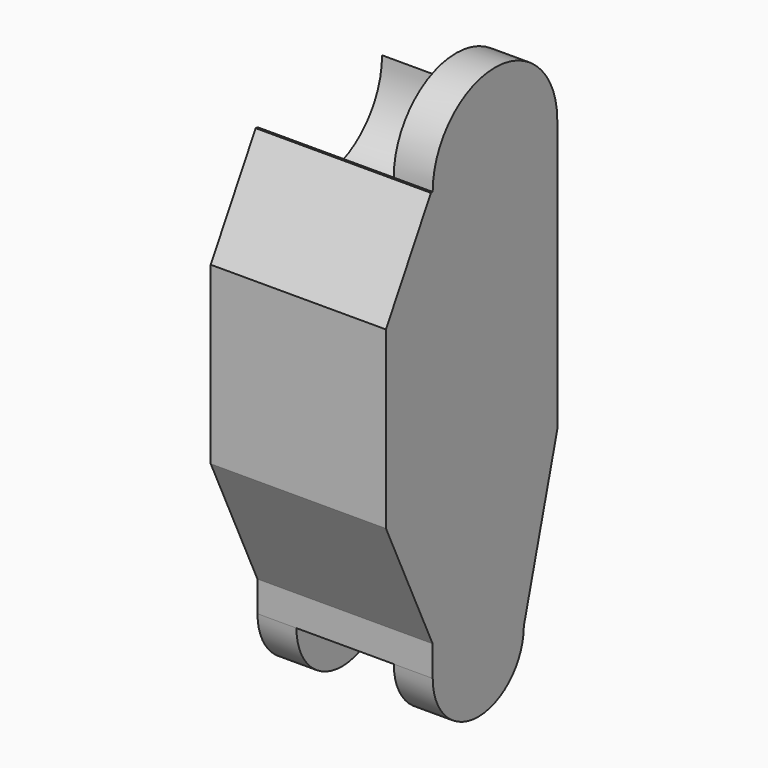
from build123d import *

# Parameters (mm, degrees)
F1_DEPTH     = 19.05
F2_DEPTH     = 114.3
F3_W         = 114.3
F3_H         = 101.6
F4_DEPTH     = 177.8
F5_T1_DEPTH  = 641.9538230647
F6_R         = 37.1475
F7_DEPTH     = 25.4
F8_R         = 37.1475
F9_DEPTH     = 25.4
F10_W        = 114.3
F10_H        = 266.7
F11_DEPTH    = 38.1
F12_T4_DEPTH = 574.9754388191
F13_T1_DEPTH = 442.85989084
F14_START    = 88.9
F14_DEPTH    = 25.4


# Not quite as in the source:
# - a fillet or chamfer that OpenCascade refuses, or shapes differently, is made with other operations: its cross-section is extruded or revolved along the edge and cut away or added


with BuildPart() as f1:
    # F0 (on Right) → F1 (new body)
    with BuildSketch(Plane.YZ):
        with BuildLine():
            Line((50.8, -101.6), (50.8, 0))
            ThreePointArc((50.8, 0), (0, -50.8), (-50.8, 0))
            Line((-50.8, 0), (-50.8, -101.6))
            Line((-50.8, -101.6), (50.8, -101.6))
        make_face()
    extrude(amount=F1_DEPTH)

    # F0 (on Right) → F2 (join)
    with BuildSketch(Plane.YZ):
        with BuildLine():
            Line((50.8, -101.6), (50.8, 0))
            ThreePointArc((50.8, 0), (0, -50.8), (-50.8, 0))
            Line((-50.8, 0), (-50.8, -101.6))
            Line((-50.8, -101.6), (50.8, -101.6))
        make_face()
    extrude(amount=F2_DEPTH)

    # F3 (on face) → F4 (join)
    with BuildSketch(Plane(origin=(0, 0, -101.6), x_dir=(1, 0, 0), z_dir=(0, 0, -1))):
        with Locations((57.15, 0)):
            Rectangle(F3_W, F3_H)
    extrude(amount=F4_DEPTH)

    # F5: chamfer of 101.6 x 27.223637951 on 1 edges, made by hand

    # F5_s2 → F5_t1 (cut)
    with BuildSketch(Plane.YZ.offset(-263.8269115324)):
        Polygon((23.576362049, -279.4), (50.8, -177.8), (50.8, -279.4), align=None)
    extrude(amount=F5_T1_DEPTH, mode=Mode.SUBTRACT)

    # F6 (on face) → F7 (join)
    with BuildSketch(Plane(origin=(0, 0, 0), x_dir=(0, -1, 0), z_dir=(-1, 0, 0))):
        with Locations((13.6118189755, -279.4)):
            Circle(F6_R)
    extrude(amount=-F7_DEPTH)

    # F8 (on face) → F9 (join)
    with BuildSketch(Plane.YZ.offset(114.3)):
        with Locations((-13.6118189755, -279.4)):
            Circle(F8_R)
    extrude(amount=-F9_DEPTH)

    # F10 (on face) → F11 (join)
    with BuildSketch(Plane.XZ.offset(50.8)):
        with Locations((57.15, -133.35)):
            Rectangle(F10_W, F10_H)
    extrude(amount=F11_DEPTH)

    # F12: chamfer of 88.9 x 41.45475081 on 1 edges, made by hand


with BuildPart() as f12_tool2:
    # F12_s3 → F12_t4 (new body)
    with BuildSketch(Plane.YZ.offset(-230.3377194096)):
        Polygon((-88.9, -177.8), (-47.44524919, -266.7), (-88.9, -266.7), align=None)
    extrude(amount=F12_T4_DEPTH)

    split(bisect_by=Plane.XZ.offset(50.8), keep=Keep.TOP)


with BuildPart() as f1_1:
    add(f1.part)

    # F12_t1: cut F12_tool2
    add(f12_tool2.part, mode=Mode.SUBTRACT)

    # F13: chamfer of 63.5 x 36.6617420935 on 1 edges, made by hand

    # F13_s2 → F13_t1 (cut)
    with BuildSketch(Plane.YZ.offset(-164.27994542)):
        Polygon((-88.9, -63.5), (-52.2382579065, 0), (-88.9, 0), align=None)
    extrude(amount=F13_T1_DEPTH, mode=Mode.SUBTRACT)

    # F0 (on Right) → F14 (join)
    with BuildSketch(Plane.YZ.offset(F14_START)):
        with BuildLine():
            Line((-50.8, 0), (50.8, 0))
            ThreePointArc((50.8, 0), (0, 50.8), (-50.8, 0))
        make_face()
        with BuildLine():
            ThreePointArc((-50.8, 0), (0, -50.8), (50.8, 0))
            Line((50.8, 0), (-50.8, 0))
        make_face()
    extrude(amount=F14_DEPTH)


solid = f1_1.part
